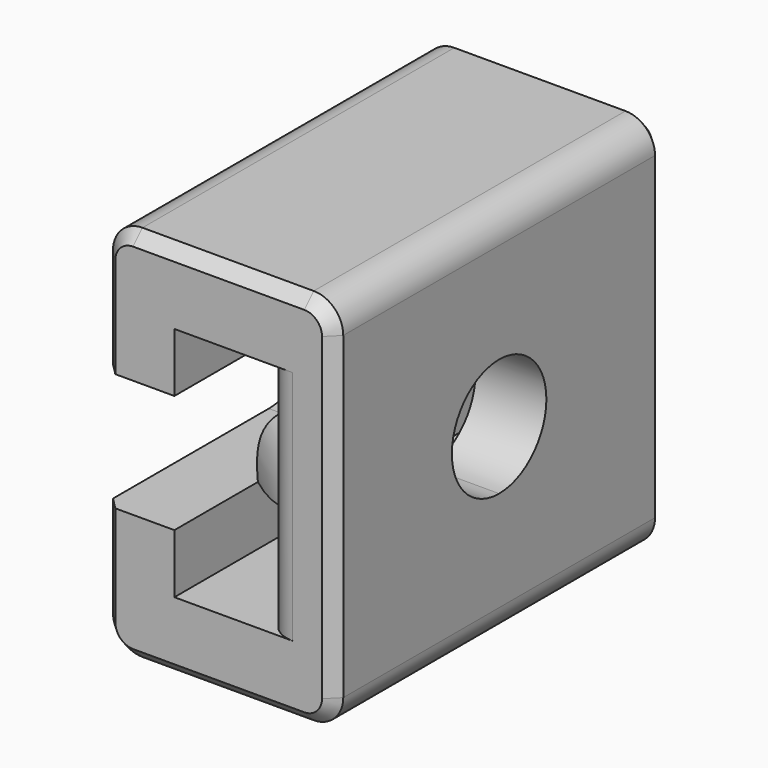
from build123d import *

# Parameters (mm, degrees)
F0_W     = 7.8
F0_H     = 12.8
F0_W_2   = 3
F0_H_2   = 8
F1_DEPTH = 14
F3_DEPTH = 7.801
F4_SIZE  = 1.99999
F5_R     = 1
F6_SIZE  = 0.4
F7_R     = 1
F8_DEPTH = 2.4


# Not quite as in the source:
# - a fillet or chamfer is up to 0.001 mm smaller than in the source, because OpenCascade refuses the exact size


with BuildPart() as f1:
    # F0 (on Front) → F1 (new body)
    with BuildSketch(Plane.XZ):
        Rectangle(F0_W, F0_H)
        Rectangle(F0_W_2, F0_H_2, mode=Mode.SUBTRACT)
    extrude(amount=F1_DEPTH)

    # F2 (on face) → F3 (cut, through all)
    with BuildSketch(Plane(origin=(-3.9, 0, 0), x_dir=(0, -1, 0), z_dir=(-1, 0, 0))):
        with BuildLine():
            Line((7, -2), (7, 2))
            ThreePointArc((7, 2), (5, 0), (7, -2))
        make_face()
        with BuildLine():
            ThreePointArc((7, -2), (8.4142135624, -1.4142135624), (9, 0))
            ThreePointArc((9, 0), (8.4142135624, 1.4142135624), (7, 2))
            Line((7, 2), (7, -2))
        make_face()
    extrude(amount=-F3_DEPTH, mode=Mode.SUBTRACT)

    # F4 (size 2 in the source; OpenCascade refuses exactly that, so slightly less here)
    f4_edges = [f1.edges().sort_by_distance(p)[0] for p in [
        (-1.5, -7, 2),
    ]]
    chamfer(f4_edges, length=F4_SIZE)

    # F5
    f5_edges = [f1.edges().sort_by_distance(p)[0] for p in [
        (3.9, -7, 6.4),
        (3.9, -7, -6.4),
        (-3.9, -7, -6.4),
        (-3.9, -7, 6.4),
    ]]
    fillet(f5_edges, radius=F5_R)

    # F6
    f6_edges = [f1.edges().sort_by_distance(p)[0] for p in [
        (3.9, -14, 0),
        (3.9, 0, 0),
    ]]
    chamfer(f6_edges, length=F6_SIZE)

    # F7
    f7_edges = [f1.edges().sort_by_distance(p)[0] for p in [
        (1.5, -14, 0),
        (1.5, 0, 0),
    ]]
    fillet(f7_edges, radius=F7_R)

    # F2 (on face) → F8 (cut, through all)
    with BuildSketch(Plane(origin=(-3.9, 0, 0), x_dir=(0, -1, 0), z_dir=(-1, 0, 0))):
        with BuildLine():
            ThreePointArc((7, 2), (8.4142135624, 1.4142135624), (9, 0))
            ThreePointArc((9, 0), (8.4142135624, -1.4142135624), (7, -2))
            Line((7, -2), (14, -2))
            Line((14, -2), (14, 2))
            Line((14, 2), (7, 2))
        make_face()
    extrude(amount=-F8_DEPTH, mode=Mode.SUBTRACT)


solid = f1.part
